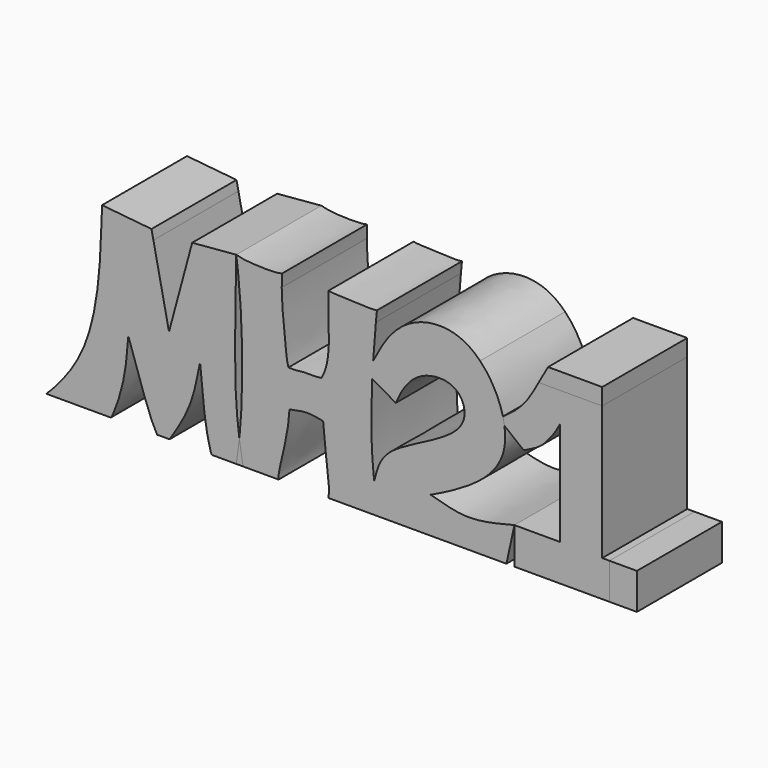
from build123d import *

# Parameters (mm, degrees)
F1_DEPTH = 25
F0_W     = 6.4472451133
F0_H     = 8.5010277107
F2_DEPTH = 25


with BuildPart() as f1:
    # F0 (on Front) → F1 (new body)
    with BuildSketch(Plane.XZ):
        with BuildLine():
            add(Edge.make_bspline(
                [(-53.2831177115, 43.3219000697), (-53.3155645531, 42.2138203548), (-53.3480113947, 41.10574064), (-53.3838228447, 40)],
                knots=[0, 0, 0, 0, 0.0560159821, 0.0560159821, 0.0560159821, 0.0560159821], degree=3))
            Line((-53.3838228447, 40), (-41.1960315485, 40))
            Line((-41.1960315485, 40), (-41.6440628469, 42.1678945422))
            Line((-41.6440628469, 42.1678945422), (-53.2831177115, 43.3219000697))
        make_face()
        with BuildLine():
            Line((-63.9121326131, 0), (-63.9121326131, 2.6014750173))
            add(Edge.make_bspline(
                [(-63.9121326131, 2.6014750173), (-65.2856485832, 1.018038843), (-66.3263440296, 0.0457523799), (-66.4394423366, 0)],
                knots=[0.8131033456, 0.8131033456, 0.8131033456, 0.8131033456, 0.9871112023, 0.9871112023, 0.9871112023, 0.9871112023], degree=3))
            Line((-66.4394423366, 0), (-63.9121326131, 0))
        make_face()
        with BuildLine():
            Line((-41.1960315485, 40), (-53.3838228447, 40))
            add(Edge.make_bspline(
                [(-53.3838228447, 40), (-53.7392436545, 29.025765953), (-54.6745805834, 14.394823164), (-62.3244435917, 4.4318172084), (-63.9121326131, 2.6014750173)],
                knots=[0.0560159821, 0.0560159821, 0.0560159821, 0.0560159821, 0.6119623544, 0.8131033456, 0.8131033456, 0.8131033456, 0.8131033456], degree=3))
            Line((-63.9121326131, 2.6014750173), (-63.9121326131, 0))
            Line((-63.9121326131, 0), (-61.9824565947, 0))
            Line((-61.9824565947, 0), (-61.1716844141, 0))
            Line((-61.1716844141, 0), (-51.3456873596, 0))
            Line((-51.3456873596, 0), (-51.2127876282, 0))
            add(Edge.make_bspline(
                [(-47.0929220319, 18.246082589), (-47.3730585954, 14.5333337163), (-47.875534313, 7.8738454639), (-50.8050580891, 0.277920138), (-51.2127876282, 0)],
                knots=[0, 0, 0, 0, 0.5260400852, 0.9435482678, 0.9435482678, 0.9435482678, 0.9435482678], degree=3))
            add(Edge.make_bspline(
                [(-47.0929220319, 18.246082589), (-45.0820892641, 12.1498495904), (-42.16266273, 3.2990368031), (-40.7536047557, 0.7830377163), (-40.3150729835, 0)],
                knots=[0, 0, 0, 0, 0.6887766294, 1, 1, 1, 1], degree=3))
            Line((-40.3150729835, 0), (-37.3912975192, 0))
            add(Edge.make_bspline(
                [(-30.2147548646, 18.246082589), (-30.8659040152, 14.8674448268), (-32.1506004624, 8.2015005883), (-35.6604280908, 2.7087478023), (-37.3912975192, 0)],
                knots=[0, 0, 0, 0, 0.5068505888, 1, 1, 1, 1], degree=3))
            add(Edge.make_bspline(
                [(-30.2147548646, 18.246082589), (-29.7748587233, 13.3151978826), (-29.0824802295, 5.554187486), (-27.7085859673, 0.19908268), (-27.4238754064, 0)],
                knots=[0, 0, 0, 0, 0.5981957208, 0.9415355428, 0.9415355428, 0.9415355428, 0.9415355428], degree=3))
            Line((-27.4238754064, 0), (-27.290975675, 0))
            Line((-27.290975675, 0), (-21.7092223465, 0))
            add(Edge.make_bspline(
                [(-20.9700228163, 5.4416856149), (-21.1593559916, 3.6191438712), (-21.4013514472, 1.8088182544), (-21.7092223465, 0)],
                knots=[0.8642577071, 0.8642577071, 0.8642577071, 0.8642577071, 1, 1, 1, 1], degree=3))
            add(Edge.make_bspline(
                [(-21.7816384355, 40), (-21.9986160572, 29.8675061984), (-22.2169329992, 16.1890134936), (-21.2743075808, 7.6378805292), (-20.9700228163, 5.4416856149)],
                knots=[0.0596058662, 0.0596058662, 0.0596058662, 0.0596058662, 0.6060648793, 0.8169290831, 0.8169290831, 0.8169290831, 0.8169290831], degree=3))
            Line((-21.7816384355, 40), (-32.7317942798, 40))
            Line((-32.7317942798, 40), (-37.5241972506, 22.2330503166))
            Line((-37.5241972506, 22.2330503166), (-41.1960315485, 40))
        make_face()
        with BuildLine():
            Line((-32.0753380656, 42.4336902797), (-32.7317942798, 40))
            Line((-32.7317942798, 40), (-21.7816384355, 40))
            add(Edge.make_bspline(
                [(-21.7092223465, 43.3219000697), (-21.7335968054, 42.2135587896), (-21.7579712642, 41.1052175095), (-21.7816384355, 40)],
                knots=[0, 0, 0, 0, 0.0596058662, 0.0596058662, 0.0596058662, 0.0596058662], degree=3))
            Line((-21.7092223465, 43.3219000697), (-32.0753380656, 42.4336902797))
        make_face()
    extrude(amount=F1_DEPTH)


with BuildPart() as f1b:
    # F0 (on Front) → F1, piece 2 (new body)
    with BuildSketch(Plane.XZ):
        with BuildLine():
            add(Edge.make_bspline(
                [(-21.7092223465, 43.3219000697), (-21.5525548563, 42.2137523734), (-21.4123914291, 41.1059798776), (-21.2872247393, 40)],
                knots=[0, 0, 0, 0, 0.0714034528, 0.0714034528, 0.0714034528, 0.0714034528], degree=3))
            Line((-21.2872247393, 40), (-11.0101087917, 40))
            add(Edge.make_bspline(
                [(-10.9431194142, 42.936515063), (-10.9943899414, 41.9091716226), (-11.0141104724, 40.9322699198), (-11.0101087917, 40)],
                knots=[0, 0, 0, 0, 0.1127929941, 0.1127929941, 0.1127929941, 0.1127929941], degree=3))
            add(Edge.make_bspline(
                [(-21.7092223465, 43.3219000697), (-19.9707277418, 42.83737728), (-16.1086546129, 42.5831461763), (-12.2224659491, 42.6191910338), (-10.9431194142, 42.936515063)],
                knots=[0, 0, 0, 0, 0.5172540084, 1, 1, 1, 1], degree=3))
        make_face()
        with BuildLine():
            add(Edge.make_bspline(
                [(0, 42.936515063), (0, 41.8916861831), (0.007397589, 40.9160183615), (0.0180792936, 40)],
                knots=[0, 0, 0, 0, 0.1076159301, 0.1076159301, 0.1076159301, 0.1076159301], degree=3))
            Line((0.0180792936, 40), (11.1388944721, 40))
            add(Edge.make_bspline(
                [(11.3866657368, 42.5625666976), (11.3012343828, 41.715728144), (11.2184982324, 40.8606927363), (11.1388944721, 40)],
                knots=[0, 0, 0, 0, 0.0518040271, 0.0518040271, 0.0518040271, 0.0518040271], degree=3))
            add(Edge.make_bspline(
                [(0, 42.936515063), (1.2794891069, 42.7011495198), (4.3349640673, 42.7538412892), (10.1586334463, 42.3332244869), (11.3866657368, 42.5625666976)],
                knots=[0, 0, 0, 0, 0.4521458666, 1, 1, 1, 1], degree=3))
        make_face()
        with BuildLine():
            Line((-11.0101087917, 40), (-21.2872247393, 40))
            add(Edge.make_bspline(
                [(-21.2872247393, 40), (-20.4925578555, 32.9782789302), (-20.1599485694, 20.8240025496), (-20.4964564264, 10.0002872051), (-20.9700228163, 5.4416856149)],
                knots=[0.0714034528, 0.0714034528, 0.0714034528, 0.0714034528, 0.5247346019, 0.8642577071, 0.8642577071, 0.8642577071, 0.8642577071], degree=3))
            add(Edge.make_bspline(
                [(-20.9700228163, 5.4416856149), (-20.7058447823, 3.5349636149), (-20.4101398326, 1.7674818074), (-20.114434883, 0)],
                knots=[0.8169290831, 0.8169290831, 0.8169290831, 0.8169290831, 1, 1, 1, 1], degree=3))
            Line((-20.114434883, 0), (-11.7471311241, 0))
            add(Edge.make_bspline(
                [(-9.1799711809, 15.3728229925), (-9.3788070779, 11.2124251112), (-11.0860332856, 4.3810850994), (-11.8155235498, 1.1136886317), (-11.7471311241, 0)],
                knots=[0, 0, 0, 0, 0.62584891, 1, 1, 1, 1], degree=3))
            add(Edge.make_bspline(
                [(-9.1799711809, 15.3728229925), (-7.5535666023, 15.7136038157), (-4.9946685175, 16.237375017), (-2.9075963583, 15.8301834987), (-1.2677678606, 15.5069287866)],
                knots=[0, 0, 0, 0, 0.5105056519, 1, 1, 1, 1], degree=3))
            add(Edge.make_bspline(
                [(-1.2677678606, 15.5069287866), (-1.0099230448, 12.0073514618), (-0.1791429191, 5.4844296415), (0.2052860238, 1.5976132491), (0, 0)],
                knots=[0, 0, 0, 0, 0.5812626367, 1, 1, 1, 1], degree=3))
            Line((0, 0), (11.3866657368, 0))
            add(Edge.make_bspline(
                [(10.7347806916, 7.0062056184), (10.9902418755, 4.5396736194), (11.2523918607, 2.2628008624), (11.3866657368, 0)],
                knots=[0.7833807096, 0.7833807096, 0.7833807096, 0.7833807096, 1, 1, 1, 1], degree=3))
            add(Edge.make_bspline(
                [(10.2811494529, 27.9978519653), (10.0488724566, 23.188500861), (9.9282574712, 15.3355372887), (10.4954210972, 9.3172733496), (10.7347806916, 7.0062056184)],
                knots=[0.2903568213, 0.2903568213, 0.2903568213, 0.2903568213, 0.5804148238, 0.7833807096, 0.7833807096, 0.7833807096, 0.7833807096], degree=3))
            Line((10.2811494529, 27.9978519653), (8.9914137498, 28.7312306464))
            add(Edge.make_bspline(
                [(8.9914137498, 28.7312306464), (9.4895275079, 29.7698073376), (9.985781339, 30.8058496054), (10.4963641495, 31.8215587649)],
                knots=[0, 0, 0, 0, 0.0473397876, 0.0473397876, 0.0473397876, 0.0473397876], degree=3))
            add(Edge.make_bspline(
                [(11.1388944721, 40), (10.8894868952, 37.3033523914), (10.6708281032, 34.5511701981), (10.4963641495, 31.8215587649)],
                knots=[0.0518040271, 0.0518040271, 0.0518040271, 0.0518040271, 0.2141118983, 0.2141118983, 0.2141118983, 0.2141118983], degree=3))
            Line((11.1388944721, 40), (0.0180792936, 40))
            add(Edge.make_bspline(
                [(0.0180792936, 40), (0.0650268859, 35.9739706129), (0.2732951968, 30.5520422531), (-0.5357871884, 26.3571533729), (-1.6412001569, 24.3313084245)],
                knots=[0.1076159301, 0.1076159301, 0.1076159301, 0.1076159301, 0.5806030613, 1, 1, 1, 1], degree=3))
            add(Edge.make_bspline(
                [(-9.4258924946, 23.9711925387), (-7.6056421312, 23.8456649349), (-6.0934590671, 24.3905923149), (-3.1436491048, 24.0540239277), (-1.6412001569, 24.3313084245)],
                knots=[0, 0, 0, 0, 0.4820750058, 1, 1, 1, 1], degree=3))
            add(Edge.make_bspline(
                [(-11.0101087917, 40), (-10.993200698, 36.0609283051), (-10.1733177224, 30.2112157712), (-9.932057782, 25.6040718922), (-9.4258924946, 23.9711925387)],
                knots=[0.1127929941, 0.1127929941, 0.1127929941, 0.1127929941, 0.5893713766, 1, 1, 1, 1], degree=3))
        make_face()
        with BuildLine():
            add(Edge.make_bspline(
                [(10.4963641495, 31.8215587649), (10.4144088468, 30.5393103312), (10.3422060056, 29.2620425803), (10.2811494529, 27.9978519653)],
                knots=[0.2141118983, 0.2141118983, 0.2141118983, 0.2141118983, 0.2903568213, 0.2903568213, 0.2903568213, 0.2903568213], degree=3))
            add(Edge.make_bspline(
                [(8.9914137498, 28.7312306464), (9.4895275079, 29.7698073376), (9.985781339, 30.8058496054), (10.4963641495, 31.8215587649)],
                knots=[0, 0, 0, 0, 0.0473397876, 0.0473397876, 0.0473397876, 0.0473397876], degree=3))
            Line((8.9914137498, 28.7312306464), (10.2811494529, 27.9978519653))
        make_face()
        with BuildLine():
            add(Edge.make_bspline(
                [(15.9833841367, 40), (16.6397168125, 40.6413222347), (21.1402942412, 44.3664500478), (29.2915421295, 45.4134356363), (34.781557836, 40.8903023758), (35.6516624522, 40)],
                knots=[0.1907966541, 0.1907966541, 0.1907966541, 0.1907966541, 0.2324412099, 0.4565017021, 0.502602279, 0.502602279, 0.502602279, 0.502602279], degree=3))
            Line((15.9833841367, 40), (35.6516624522, 40))
        make_face()
        with BuildLine():
            Line((35.6516624522, 40), (15.9833841367, 40))
            add(Edge.make_bspline(
                [(10.4963641495, 31.8215587649), (12.043616762, 34.8995289164), (13.7224540539, 37.7907777766), (15.9833841367, 40)],
                knots=[0.0473397876, 0.0473397876, 0.0473397876, 0.0473397876, 0.1907966541, 0.1907966541, 0.1907966541, 0.1907966541], degree=3))
            add(Edge.make_bspline(
                [(10.4963641495, 31.8215587649), (10.4144088468, 30.5393103312), (10.3422060056, 29.2620425803), (10.2811494529, 27.9978519653)],
                knots=[0.2141118983, 0.2141118983, 0.2141118983, 0.2141118983, 0.2903568213, 0.2903568213, 0.2903568213, 0.2903568213], degree=3))
            Line((10.2811494529, 27.9978519653), (15.8307757229, 24.842184037))
            add(Edge.make_bspline(
                [(15.8307757229, 24.842184037), (17.2759995512, 28.3164145311), (20.7188361179, 33.4142248279), (30.9934005445, 33.9475891373), (34.2427776007, 22.6343096552), (12.2709515136, 15.7806768546), (11.4232382084, 9.3539075188), (10.7347806916, 7.0062056184)],
                knots=[0, 0, 0, 0, 0.1948756979, 0.3729823275, 0.5415594818, 0.8226775477, 1, 1, 1, 1], degree=3))
            add(Edge.make_bspline(
                [(10.7347806916, 7.0062056184), (10.9902418755, 4.5396736194), (11.2523918607, 2.2628008624), (11.3866657368, 0)],
                knots=[0.7833807096, 0.7833807096, 0.7833807096, 0.7833807096, 1, 1, 1, 1], degree=3))
            Line((11.3866657368, 0), (12.7463592216, 0))
            Line((12.7463592216, 0), (41.847165674, 0))
            Line((41.847165674, 0), (43.7246337533, 8.6154667661))
            add(Edge.make_bspline(
                [(24.0111835301, 8.4813619033), (27.2843466993, 7.6443603037), (32.5842292631, 5.8274313376), (39.8816469953, 7.6406623418), (43.7246337533, 8.6154667661)],
                knots=[0, 0, 0, 0, 0.4716444986, 1, 1, 1, 1], degree=3))
            add(Edge.make_bspline(
                [(41.3834220736, 28.4180595906), (41.6214590829, 26.7640241509), (41.5794161521, 17.7562777998), (32.4651177029, 12.5184818216), (24.0111835301, 8.4813619033)],
                knots=[0.6587329187, 0.6587329187, 0.6587329187, 0.6587329187, 0.7203278409, 1, 1, 1, 1], degree=3))
            Line((41.3834220736, 28.4180595906), (39.9696938694, 29.5358616859))
            add(Edge.make_bspline(
                [(39.9696938694, 29.5358616859), (40.3388372194, 29.7728350062), (40.6910433479, 30.004744341), (41.0277565553, 30.2329677509)],
                knots=[0, 0, 0, 0, 0.0549869476, 0.0549869476, 0.0549869476, 0.0549869476], degree=3))
            add(Edge.make_bspline(
                [(35.6516624522, 40), (38.1748380835, 37.4182538314), (40.1369755289, 33.840275622), (41.0277565553, 30.2329677509)],
                knots=[0.502602279, 0.502602279, 0.502602279, 0.502602279, 0.636287183, 0.636287183, 0.636287183, 0.636287183], degree=3))
        make_face()
        with BuildLine():
            add(Edge.make_bspline(
                [(41.0277565553, 30.2329677509), (41.1773189588, 29.6272996697), (41.2966792768, 29.0208047703), (41.3834220736, 28.4180595906)],
                knots=[0.636287183, 0.636287183, 0.636287183, 0.636287183, 0.6587329187, 0.6587329187, 0.6587329187, 0.6587329187], degree=3))
            add(Edge.make_bspline(
                [(39.9696938694, 29.5358616859), (40.3388372194, 29.7728350062), (40.6910433479, 30.004744341), (41.0277565553, 30.2329677509)],
                knots=[0, 0, 0, 0, 0.0549869476, 0.0549869476, 0.0549869476, 0.0549869476], degree=3))
            Line((39.9696938694, 29.5358616859), (41.3834220736, 28.4180595906))
        make_face()
    extrude(amount=F1_DEPTH)


with BuildPart() as f1c:
    # F0 (on Front) → F1, piece 3 (new body)
    with BuildSketch(Plane.XZ):
        with BuildLine():
            add(Edge.make_bspline(
                [(49.4192727713, 40), (50.1185268473, 41.2879822775), (50.8355057851, 42.6193901592), (51.6427792609, 43.9200587571)],
                knots=[0.7694557398, 0.7694557398, 0.7694557398, 0.7694557398, 1, 1, 1, 1], degree=3))
            Line((49.4192727713, 40), (64.3768236041, 40))
            Line((64.3768236041, 40), (64.3768236041, 43.9200587571))
            Line((64.3768236041, 43.9200587571), (51.6427792609, 43.9200587571))
        make_face()
    extrude(amount=F1_DEPTH)


with BuildPart() as f1d:
    # F0 (on Front) → F1, piece 4 (new body)
    with BuildSketch(Plane.XZ):
        with Locations((69.3114899435, 4.2505138554)):
            Rectangle(F0_W, F0_H)
    extrude(amount=F1_DEPTH)


with BuildPart() as f2:
    # F0 (on Front) → F2 (new body)
    with BuildSketch(Plane.XZ):
        with BuildLine():
            Line((64.3768236041, 40), (49.4192727713, 40))
            add(Edge.make_bspline(
                [(41.0277565553, 30.2329677509), (43.7435642968, 32.073735769), (46.4949594137, 34.6528535545), (48.5974237979, 38.4862055882), (49.4192727713, 40)],
                knots=[0.0549869476, 0.0549869476, 0.0549869476, 0.0549869476, 0.4984919083, 0.7694557398, 0.7694557398, 0.7694557398, 0.7694557398], degree=3))
            add(Edge.make_bspline(
                [(41.0277565553, 30.2329677509), (41.1773189588, 29.6272996697), (41.2966792768, 29.0208047703), (41.3834220736, 28.4180595906)],
                knots=[0.636287183, 0.636287183, 0.636287183, 0.636287183, 0.6587329187, 0.6587329187, 0.6587329187, 0.6587329187], degree=3))
            Line((41.3834220736, 28.4180595906), (45.930031687, 24.8231608421))
            add(Edge.make_bspline(
                [(45.930031687, 24.8231608421), (49.2474734537, 26.36328751), (50.8217337037, 27.6417450729), (53.542861599, 31.1566749984), (54.4175393879, 32.9842269421)],
                knots=[0, 0, 0, 0, 0.5103697239, 1, 1, 1, 1], degree=3))
            Line((54.4175393879, 32.9842269421), (54.4175393879, 8.6154667661))
            Line((54.4175393879, 8.6154667661), (43.7246337533, 8.6154667661))
            Line((43.7246337533, 8.6154667661), (43.7246337533, 0))
            Line((43.7246337533, 0), (66.0878673869, 0))
            Line((66.0878673869, 0), (66.0878673869, 8.5010277107))
            Line((66.0878673869, 8.5010277107), (64.3768236041, 8.5010277107))
            Line((64.3768236041, 8.5010277107), (64.3768236041, 40))
        make_face()
    extrude(amount=F2_DEPTH)


with BuildPart() as f2b:
    # F0 (on Front) → F2, piece 2 (new body)
    with BuildSketch(Plane.XZ):
        with BuildLine():
            add(Edge.make_bspline(
                [(-20.9700228163, 5.4416856149), (-20.7058447823, 3.5349636149), (-20.4101398326, 1.7674818074), (-20.114434883, 0)],
                knots=[0.8169290831, 0.8169290831, 0.8169290831, 0.8169290831, 1, 1, 1, 1], degree=3))
            add(Edge.make_bspline(
                [(-20.9700228163, 5.4416856149), (-21.1593559916, 3.6191438712), (-21.4013514472, 1.8088182544), (-21.7092223465, 0)],
                knots=[0.8642577071, 0.8642577071, 0.8642577071, 0.8642577071, 1, 1, 1, 1], degree=3))
            Line((-21.7092223465, 0), (-20.114434883, 0))
        make_face()
    extrude(amount=F2_DEPTH)


solid = Compound([f1.part, f1b.part, f1c.part, f1d.part, f2.part, f2b.part])
